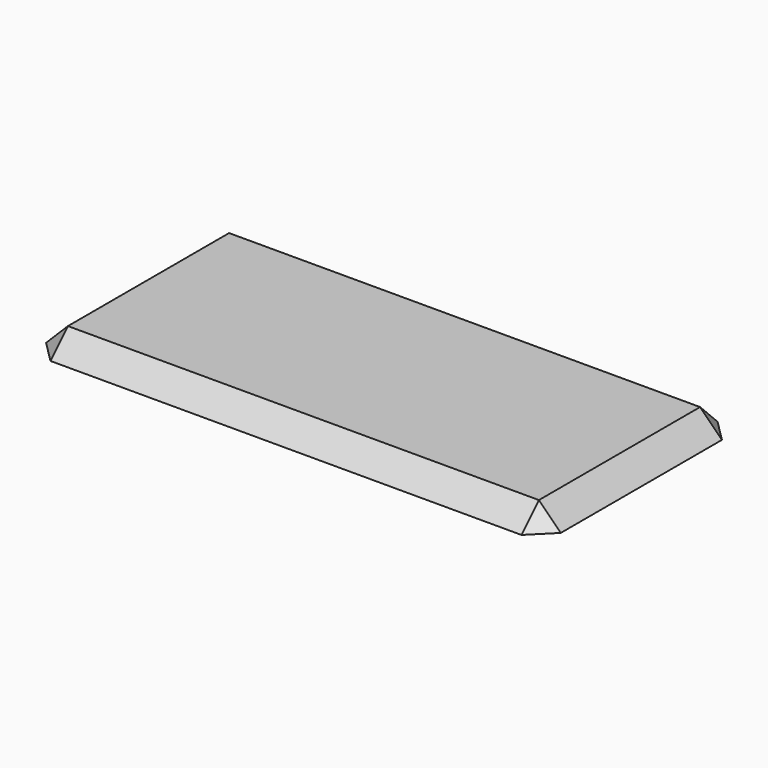
from build123d import *

# Parameters (mm, degrees)
F0_W     = 47.8917
F0_H     = 22.8092
F1_DEPTH = 2.032
F2_SIZE  = 2.03199


# Not quite as in the source:
# - a fillet or chamfer is up to 0.001 mm smaller than in the source, because OpenCascade refuses the exact size


with BuildPart() as f1:
    # F0 (on Top) → F1 (new body)
    with BuildSketch(Plane.XY):
        Rectangle(F0_W, F0_H)
    extrude(amount=F1_DEPTH)

    # F2 (size 2.032 in the source; OpenCascade refuses exactly that, so slightly less here)
    f2_edges = [f1.edges().sort_by_distance(p)[0] for p in [
        (0, -11.4046, 2.032),
        (-23.94585, 0, 2.032),
        (0, 11.4046, 2.032),
        (23.94585, 0, 2.032),
        (23.94585, -11.4046, 1.016),
        (-23.94585, -11.4046, 1.016),
        (23.94585, 11.4046, 1.016),
        (-23.94585, 11.4046, 1.016),
    ]]
    chamfer(f2_edges, length=F2_SIZE)


solid = f1.part
